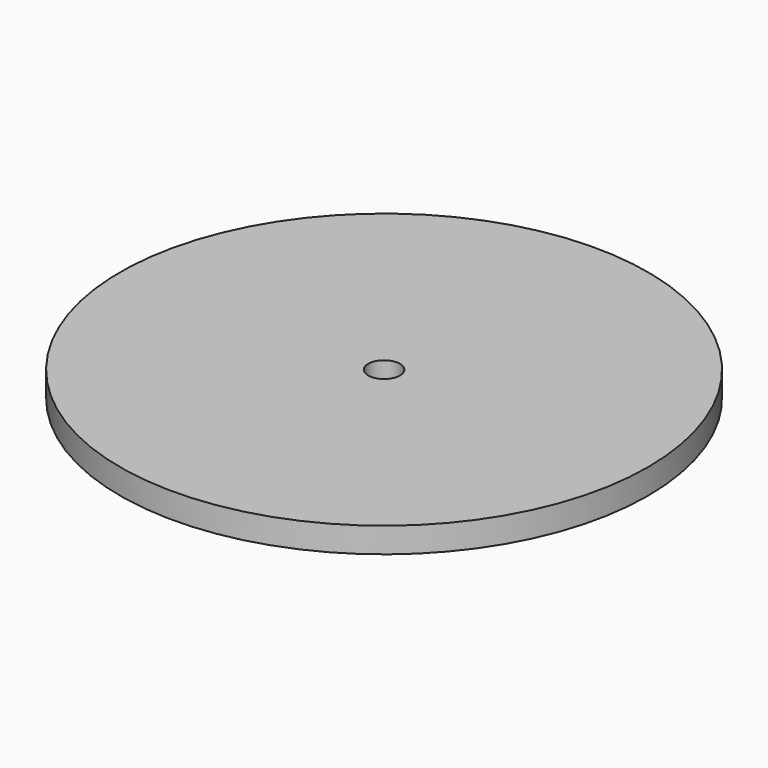
from build123d import *

# Parameters (mm, degrees)
F0_R     = 49.873
F0_R_2   = 3
F1_DEPTH = 4.7625


# Not quite as in the source:
# - a length typed as a fraction of an inch, garbled in the dataset ("3 / 203.2 mm" for 3/8 in), is restored


with BuildPart() as f1:
    # F0 (on Top) → F1 (new body)
    with BuildSketch(Plane.XY):
        Circle(F0_R)
        Circle(F0_R_2, mode=Mode.SUBTRACT)
    extrude(amount=F1_DEPTH)


solid = f1.part
